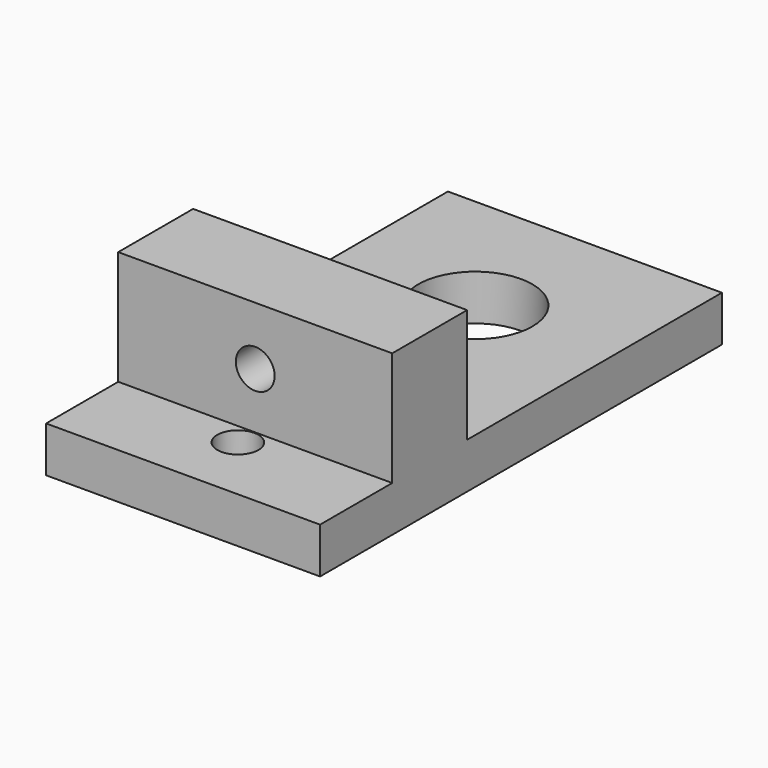
from build123d import *

# Parameters (mm, degrees)
F0_W     = 12
F0_H     = 4.1
F1_DEPTH = 7
F0_H_2   = 13.95
F0_R     = 0.9
F0_R_2   = 4
F0_H_3   = 3.95
F0_R_3   = 2.5
F2_DEPTH = 2
F4_R     = 0.85
F5_DEPTH = 5


# Not quite as in the source:
# - a feature of the source that left no trace in its solid (it failed there, or was rolled back) is left out


with BuildPart() as f1:
    # F0 (on Top) → F1 (new body)
    with BuildSketch(Plane.XY):
        with Locations((-0.3663106412, 0)):
            Rectangle(F0_W, F0_H)
    extrude(amount=F1_DEPTH)

    # F0 (on Top) → F2 (join)
    with BuildSketch(Plane.XY):
        with Locations((-0.3663106412, 9.025)):
            Rectangle(F0_W, F0_H_2)
        with Locations((-0.3663106412, 3)):
            Circle(F0_R, mode=Mode.SUBTRACT)
        with Locations((-0.3663106412, 10)):
            Circle(F0_R_2, mode=Mode.SUBTRACT)
        with Locations((-0.3663106412, -4.025)):
            Rectangle(F0_W, F0_H_3)
        with Locations((-0.3663106412, -3)):
            Circle(F0_R, mode=Mode.SUBTRACT)
        with Locations((-0.3663106412, 10)):
            Circle(F0_R_2)
        with Locations((-0.3663106412, 10)):
            Circle(F0_R_3, mode=Mode.SUBTRACT)
    extrude(amount=F2_DEPTH)

    # F4 (on face) → F5 (cut)
    with BuildSketch(Plane(origin=(0, 2.05, 0), x_dir=(-1, 0, 0), z_dir=(0, 1, 0))):
        with Locations((0.3663106412, 4.45)):
            Circle(F4_R)
    extrude(amount=-F5_DEPTH, mode=Mode.SUBTRACT)


solid = f1.part
